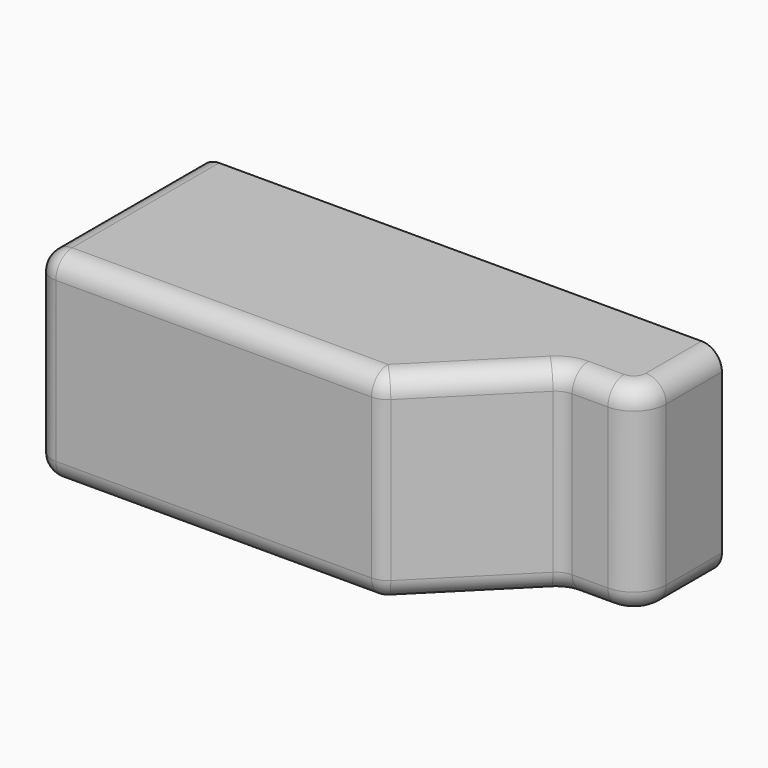
from build123d import *

# Parameters (mm, degrees)
F0_W     = 111.1538112164
F0_H     = 49.8025715351
F1_DEPTH = 50.8
F2_R     = 5.08
F3_SIZE  = 25.4
F4_W     = 25.4
F4_H     = 49.8025715351
F5_DEPTH = 19.05
F6_R     = 8.0573195259
F7_F1_R  = 5.08
F7_F2_R  = 5.08
F7_F3_R  = 5.08
F7_F4_R  = 5.08


# Not quite as in the source:
# - a feature of the source that left no trace in its solid (it failed there, or was rolled back) is left out


with BuildPart() as f1:
    # F0 (on Front) → F1 (new body)
    with BuildSketch(Plane.XZ):
        Rectangle(F0_W, F0_H)
    extrude(amount=F1_DEPTH)

    # F2
    f2_edges = [f1.edges().sort_by_distance(p)[0] for p in [
        (-55.576906, -50.8, 0),
    ]]
    fillet(f2_edges, radius=F2_R)

    # F3
    f3_edges = [f1.edges().sort_by_distance(p)[0] for p in [
        (55.576906, -50.8, 0),
    ]]
    chamfer(f3_edges, length=F3_SIZE)

    # F4 (on face) → F5 (join)
    with BuildSketch(Plane.YZ.offset(55.5769056082)):
        with Locations((-12.7, 0)):
            Rectangle(F4_W, F4_H)
    extrude(amount=F5_DEPTH)

    # F6
    f6_edges = [f1.edges().sort_by_distance(p)[0] for p in [
        (74.626906, -25.4, 0),
    ]]
    fillet(f6_edges, radius=F6_R)

    # F7: fillet of radius 5.08 on 4 edges, made by hand

    # F7_f1
    f7_f1_edges = [f1.edges().sort_by_distance(p)[0] for p in [
        (55.5769056082, -25.4, 0),
    ]]
    fillet(f7_f1_edges, radius=F7_F1_R)

    # F7_f2
    f7_f2_edges = [f1.edges().sort_by_distance(p)[0] for p in [
        (30.1769056082, -50.8, 0),
    ]]
    fillet(f7_f2_edges, radius=F7_F2_R)

    # F7_f3
    f7_f3_edges = [f1.edges().sort_by_distance(p)[0] for p in [
        (42.8769056082, -38.1, 24.9012857676),
    ]]
    fillet(f7_f3_edges, radius=F7_F3_R)

    # F7_f4
    f7_f4_edges = [f1.edges().sort_by_distance(p)[0] for p in [
        (42.8769056082, -38.1, -24.9012857676),
    ]]
    fillet(f7_f4_edges, radius=F7_F4_R)


solid = f1.part
